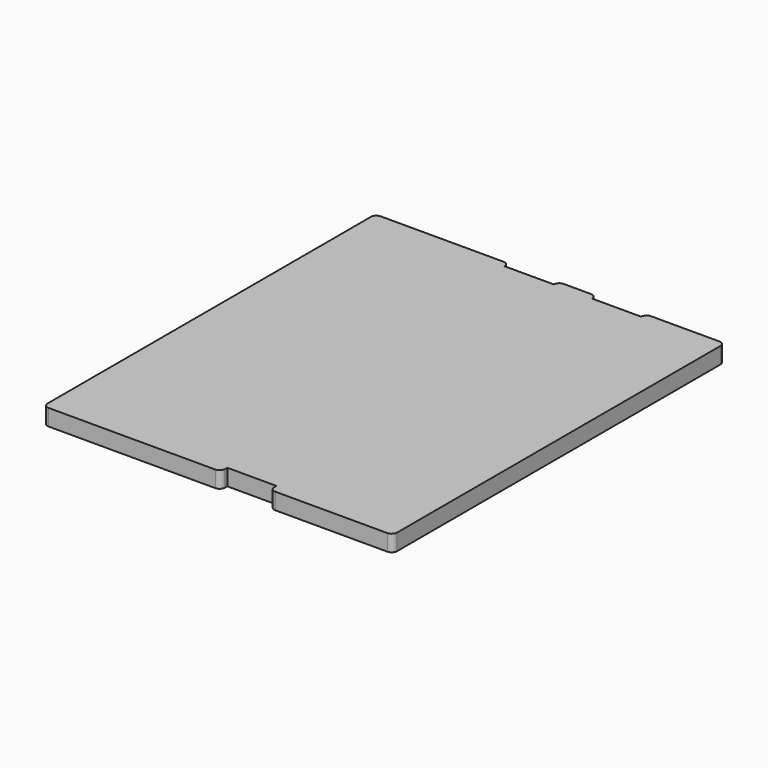
from build123d import *

# Parameters (mm, degrees)
F0_W     = 203.2
F0_H     = 241.3
F1_DEPTH = 9.525
F2_W     = 28.575
F2_H     = 9.525
F3_DEPTH = 4.7625
F4_W     = 28.575
F4_H     = 9.525
F5_DEPTH = 3.175
F6_R     = 3.17499


# Not quite as in the source:
# - a fillet or chamfer is up to 0.001 mm smaller than in the source, because OpenCascade refuses the exact size


with BuildPart() as f1:
    # F0 (on Top) → F1 (new body)
    with BuildSketch(Plane.XY):
        Rectangle(F0_W, F0_H)
    extrude(amount=F1_DEPTH)

    # F2 (on face) → F3 (cut)
    with BuildSketch(Plane.XZ.offset(120.65)):
        with Locations((15.875, 4.7625)):
            Rectangle(F2_W, F2_H)
    extrude(amount=-F3_DEPTH, mode=Mode.SUBTRACT)

    # F4 (on face) → F5 (cut)
    with BuildSketch(Plane(origin=(0, 120.65, 0), x_dir=(-1, 0, 0), z_dir=(0, 1, 0))):
        with Locations((-41.275, 4.7625)):
            Rectangle(F4_W, F4_H)
        with Locations((9.525, 4.7625)):
            Rectangle(F4_W, F4_H)
    extrude(amount=-F5_DEPTH, mode=Mode.SUBTRACT)

    # F6 (radius 3.175 in the source; OpenCascade refuses exactly that, so slightly less here)
    f6_edges = [f1.edges().sort_by_distance(p)[0] for p in [
        (-101.6, 120.65, 4.7625),
        (-23.8125, 120.65, 4.7625),
        (4.7625, 120.65, 4.7625),
        (26.9875, 120.65, 4.7625),
        (55.5625, 120.65, 4.7625),
        (101.6, 120.65, 4.7625),
        (-101.6, -120.65, 4.7625),
        (1.5875, -120.65, 4.7625),
        (30.1625, -120.65, 4.7625),
        (101.6, -120.65, 4.7625),
    ]]
    fillet(f6_edges, radius=F6_R)


solid = f1.part
